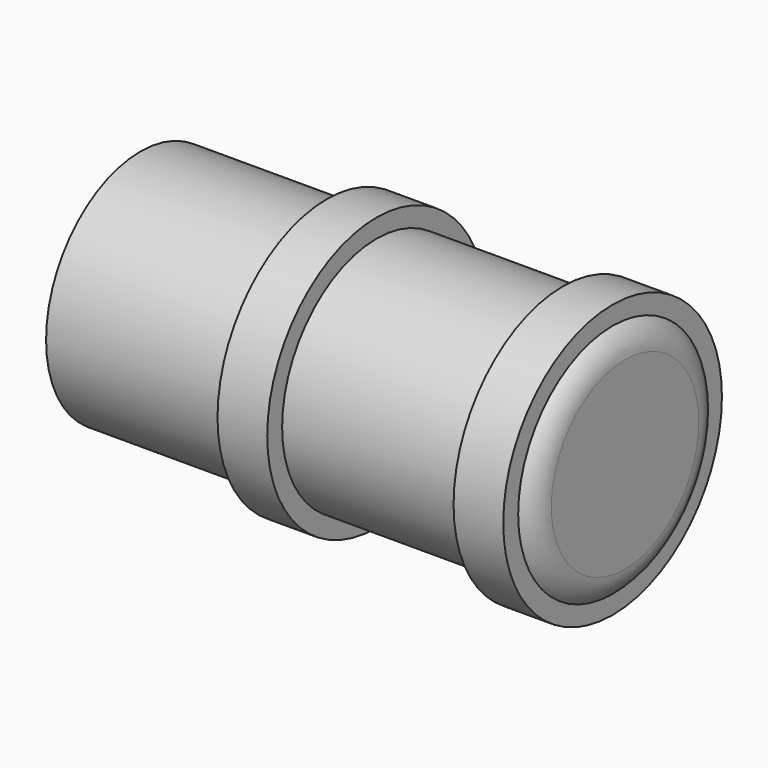
from build123d import *

# Parameters (mm, degrees)
F0_R      = 9.5
F1_DEPTH  = 15
F2_R      = 11
F3_DEPTH  = 4
F4_R      = 9.5
F5_DEPTH  = 15
F6_R      = 11
F7_DEPTH  = 4
F8_R      = 9.5
F9_DEPTH  = 1
F11_R     = 8.65
F12_DEPTH = 36.3
F15_DEPTH = 0.5
F16_DEPTH = 0.5


# Not quite as in the source:
# - a fillet or chamfer that OpenCascade refuses, or shapes differently, is made with other operations: its cross-section is extruded or revolved along the edge and cut away or added


with BuildPart() as f1:
    # F0 (on Right) → F1 (new body)
    with BuildSketch(Plane.YZ):
        Circle(F0_R)
    extrude(amount=F1_DEPTH)

    # F2 (on face) → F3 (join)
    with BuildSketch(Plane.YZ.offset(15)):
        Circle(F2_R)
    extrude(amount=F3_DEPTH)

    # F4 (on face) → F5 (join)
    with BuildSketch(Plane.YZ.offset(19)):
        Circle(F4_R)
    extrude(amount=F5_DEPTH)

    # F6 (on face) → F7 (join)
    with BuildSketch(Plane.YZ.offset(34)):
        Circle(F6_R)
    extrude(amount=F7_DEPTH)

    # F8 (on face) → F9 (join)
    with BuildSketch(Plane.YZ.offset(38)):
        Circle(F8_R)
    extrude(amount=F9_DEPTH)

    # F10: fillet of radius 2.6556349186 on 1 edges, made by hand

    # F10_s1 → F10_t2 (revolve, cut)
    with BuildSketch(Plane.XY):
        with BuildLine():
            ThreePointArc((38, 9.5), (38.7369744021, 8.5759498633), (39, 7.4236402438))
            Line((39, 7.4236402438), (39, 9.5))
            Line((39, 9.5), (38, 9.5))
        make_face()
    revolve(axis=Axis((39, 0, 0), (1, 0, 0)), mode=Mode.SUBTRACT)

    # F11 (on face) → F12 (cut)
    with BuildSketch(Plane(origin=(0, 0, 0), x_dir=(0, -1, 0), z_dir=(-1, 0, 0))):
        Circle(F11_R)
    extrude(amount=-F12_DEPTH, mode=Mode.SUBTRACT)

    # F14 (on Front) → F15 (join, symmetric)
    with BuildSketch(Plane.XZ):
        Polygon((25.5720777049, -8.6574743293), (25.5720777049, 8.6425256707), (24.0004413285, 7.0708892943), (22.4288049522, 8.6425256707), (22.4288049522, -8.6574743293), (24.0004413285, -7.085837953), align=None)
    extrude(amount=F15_DEPTH, both=True)

    # F13 (on Top) → F16 (join, symmetric)
    with BuildSketch(Plane.XY):
        Polygon((24.1439803634, 5.9105833968), (22.2261317603, 8.5902402711), (22.2261317603, -8.7097597289), (24.1439803634, -6.0301028546), (26.0618289666, -8.7097597289), (26.0618289666, 8.5902402711), align=None)
    extrude(amount=F16_DEPTH, both=True)


solid = f1.part
